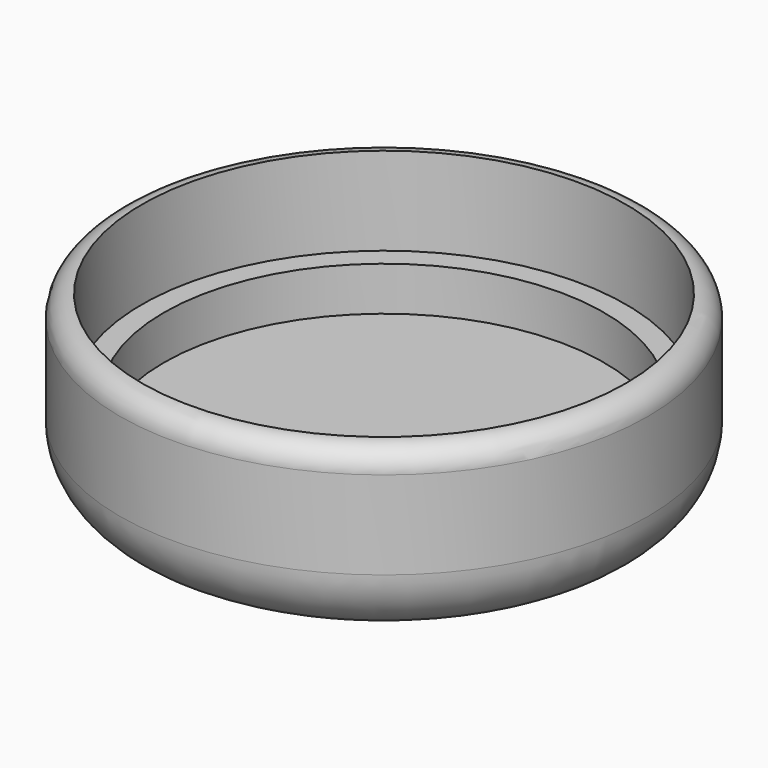
from build123d import *

# Parameters (mm, degrees)
F0_R     = 12
F1_DEPTH = 8
F2_R     = 10
F3_DEPTH = 6
F2_R_2   = 11
F4_DEPTH = 4
F5_R     = 3
F6_R     = 0.99999


# Not quite as in the source:
# - a fillet or chamfer is up to 0.001 mm smaller than in the source, because OpenCascade refuses the exact size


with BuildPart() as f1:
    # F0 (on Top) → F1 (new body)
    with BuildSketch(Plane.XY):
        Circle(F0_R)
    extrude(amount=F1_DEPTH)

    # F2 (on face) → F3 (cut)
    with BuildSketch(Plane.XY.offset(8)):
        Circle(F2_R)
    extrude(amount=-F3_DEPTH, mode=Mode.SUBTRACT)

    # F2 (on face) → F4 (cut)
    with BuildSketch(Plane.XY.offset(8)):
        Circle(F2_R_2)
        Circle(F2_R, mode=Mode.SUBTRACT)
    extrude(amount=-F4_DEPTH, mode=Mode.SUBTRACT)

    # F5
    f5_edges = [f1.edges().sort_by_distance(p)[0] for p in [
        (-12, 0, 0),
    ]]
    fillet(f5_edges, radius=F5_R)

    # F6 (radius 1 in the source; OpenCascade refuses exactly that, so slightly less here)
    f6_edges = [f1.edges().sort_by_distance(p)[0] for p in [
        (-12, 0, 8),
    ]]
    fillet(f6_edges, radius=F6_R)


solid = f1.part
